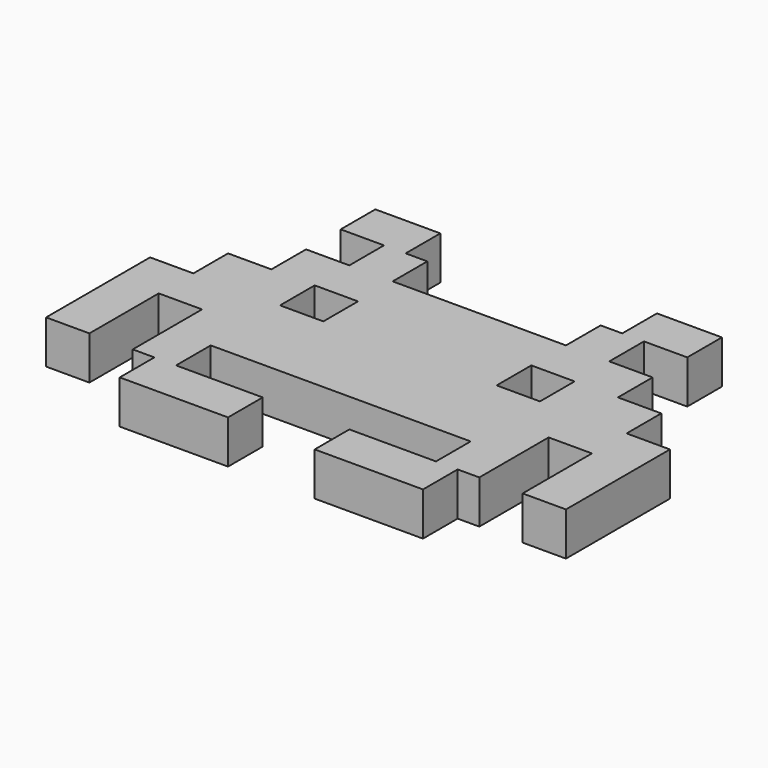
from build123d import *

# Parameters (mm, degrees)
F0_W     = 10
F0_H     = 10
F0_R     = 6
F1_DEPTH = 10
F3_DEPTH = 3


with BuildPart() as f1:
    # F0 (on Top) → F1 (new body)
    with BuildSketch(Plane.XY):
        Polygon((10, 0), (0, 0), (-10, 0), (-20, 0), (-20, 10), (-25, 10), (-30, 10), (-30, 0), (-40, 0), (-40, -10), (-50, -10), (-50, -20), (-60, -20), (-60, -30), (-60, -50), (-50, -50), (-50, -30), (-40, -30), (-40, -40), (-40, -50), (-35, -50), (-30, -50), (-30, -40), (-20, -40), (-10, -40), (0, -40), (10, -40), (20, -40), (30, -40), (30, -50), (35, -50), (40, -50), (40, -40), (40, -30), (50, -30), (50, -50), (60, -50), (60, -30), (60, -20), (50, -20), (50, -10), (40, -10), (40, 0), (30, 0), (30, 10), (25, 10), (20, 10), (20, 0), align=None)
        with Locations((-25, -15)):
            Rectangle(F0_W, F0_H, mode=Mode.SUBTRACT)
        with Locations((0, -12)):
            Circle(F0_R, mode=Mode.SUBTRACT)
        with Locations((25, -15)):
            Rectangle(F0_W, F0_H, mode=Mode.SUBTRACT)
        Polygon((-30, 10), (-25, 10), (-25, 20), (-30, 20), (-40, 20), (-40, 10), align=None)
        Polygon((25, 20), (25, 10), (30, 10), (40, 10), (40, 20), (30, 20), align=None)
        Polygon((-30, -50), (-35, -50), (-35, -60), (-10, -60), (-10, -50), align=None)
        Polygon((35, -60), (35, -50), (30, -50), (10, -50), (10, -60), align=None)
        with Locations((0, -12)):
            Circle(F0_R)
    extrude(amount=F1_DEPTH)

    # F2 (on Right) → F3 (cut, symmetric)
    with BuildSketch(Plane.YZ):
        Polygon((-10, 5), (-10, 0), (-4, 0), (-1.1132486541, 5), align=None)
    extrude(amount=F3_DEPTH, both=True, mode=Mode.SUBTRACT)


solid = f1.part
